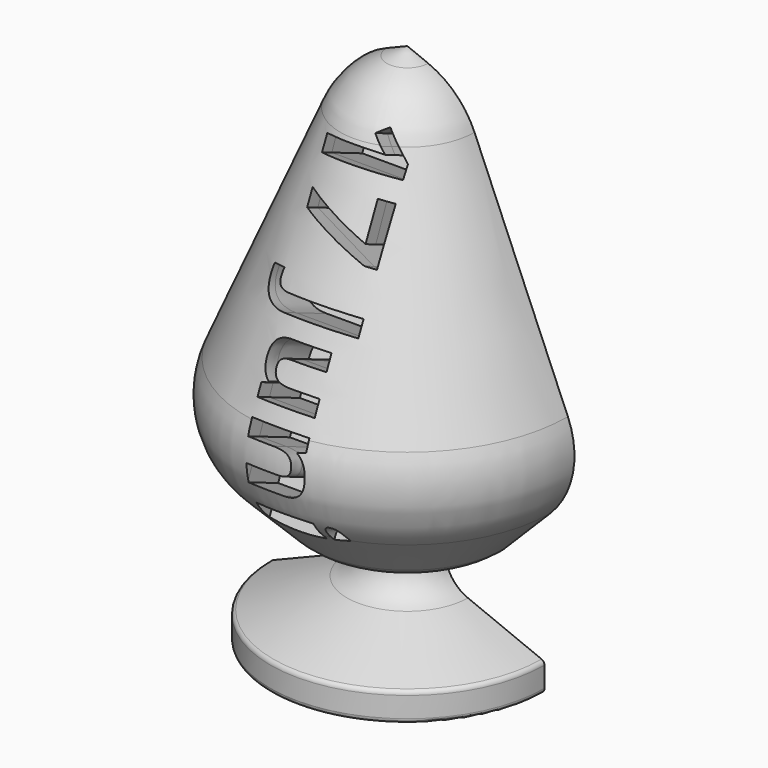
from build123d import *

# Parameters (mm, degrees)
F1_ANGLE_BACK = 90
F1_ANGLE      = 180
F4_TEXT_SIZE  = 25.4063142163
F5_DEPTH      = 10
F5_DEPTH_BACK = 25


# Not quite as in the source:
# - Text() gives the source's letters only with a copy of the font that has no kerning and outlines rounded to 1/6400 em; it was checked with that copy


with BuildPart() as f1:
    # F0 (on Right) → F1 (revolve)
    with BuildSketch(Plane.YZ, mode=Mode.PRIVATE) as f1_sk:
        with BuildLine():
            Line((0, -22.5338969827), (0, 104.4661030173))
            Line((0, 104.4661030173), (-5.0110840239, 102.4255827069))
            ThreePointArc((-5.0110840239, 102.4255827069), (-11.7076244231, 98.0155318736), (-16.2158115918, 91.3846608808))
            Line((-16.2158115918, 91.3846608808), (-38.7806370854, 38.2252633572))
            ThreePointArc((-38.7806370854, 38.2252633572), (-40.0065285663, 26.6122261617), (-34.5382443623, 16.2941201974))
            Line((-34.5382443623, 16.2941201974), (-23.3812653679, 5.0966881688))
            ThreePointArc((-23.3812653679, 5.0966881688), (-20.6661564507, 3.1597229321), (-17.465083791, 2.2233551687))
            Line((-17.465083791, 2.2233551687), (-9.9063044495, 1.3346594563))
            ThreePointArc((-9.9063044495, 1.3346594563), (-9.3277186827, 1.0330923116), (-9.0957742182, 0.4232513506))
            Line((-9.0957742182, 0.4232513506), (-9.0957742182, 0))
            ThreePointArc((-9.0957742182, 0), (-10.6035031728, -4.9410229563), (-14.6129649164, -8.1985021936))
            Line((-14.6129649164, -8.1985021936), (-32.4237018781, -15.4389329408))
            ThreePointArc((-32.4237018781, -15.4389329408), (-32.9334192459, -15.8530518048), (-33.1250947583, -16.4811972709))
            Line((-33.1250947583, -16.4811972709), (-33.1250947583, -21.4088022243))
            ThreePointArc((-33.1250947583, -21.4088022243), (-32.7955621331, -22.2043643574), (-32, -22.5338969827))
            Line((-32, -22.5338969827), (0, -22.5338969827))
        make_face()
    revolve(f1_sk.sketch.rotate(Axis((0, 0, 13.0628068), (0, 0, -1)), -F1_ANGLE_BACK), axis=Axis((0, 0, 13.0628068), (0, 0, -1)), revolution_arc=F1_ANGLE)

    # F4 (on line) → F5 (cut, two sides)
    with BuildSketch(Plane(origin=(0, -42.4130383338, 18.0127657761), x_dir=(1, 0, 0), z_dir=(0, -0.9204306923, 0.3909057951))) as f5_sk:
        with Locations(Location((-7.1465927951, 83.4300683075), (0, 0, -90))):
            Text('17 Juni', F4_TEXT_SIZE, font='Open Sans', font_style=FontStyle.BOLD, text_align=(TextAlign.LEFT, TextAlign.BOTTOM))
    extrude(amount=-F5_DEPTH, mode=Mode.SUBTRACT)
    extrude(f5_sk.sketch, amount=F5_DEPTH_BACK, mode=Mode.SUBTRACT)


solid = f1.part
